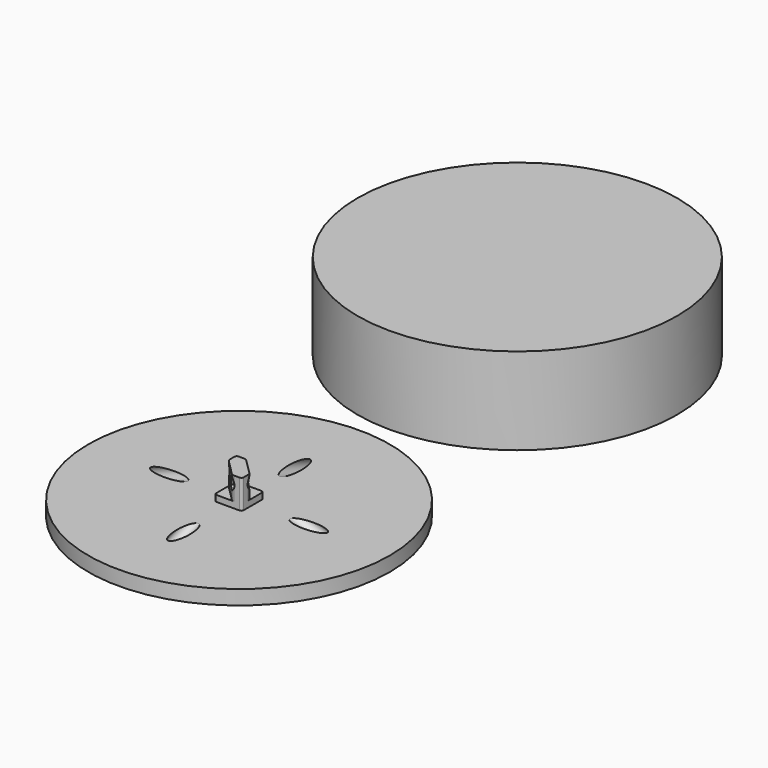
from build123d import *

# Parameters (mm, degrees)
F0_R              = 16.51
F1_DEPTH          = 1.5875
F2_W              = 3
F2_H              = 3
F3_DEPTH          = 3.175
F9_DEPTH          = 2.5
F10_R             = 17.5006
F11_DEPTH         = 9.525
F16_R             = 0.7
F17_DEPTH         = 1.27
F17_COPIES2_COUNT = 2
F18_DEPTH         = 25.4
F18_COPIES_COUNT  = 4
F19_R             = 0.254
F20_R             = 0.508


# Not quite as in the source:
# - a length typed as a fraction of an inch, garbled in the dataset ("3 / 203.2 mm" for 3/8 in), is restored
# - a pattern or mirror of a feature is missing from the dataset's text; its kind, count and spacing are read off the source's solid


with BuildPart() as f1:
    # F0 (on Top) → F1 (new body)
    with BuildSketch(Plane.XY):
        Circle(F0_R)
    extrude(amount=F1_DEPTH)

    # F2 (on face) → F3 (join)
    with BuildSketch(Plane.XY.offset(1.5875)):
        Rectangle(F2_W, F2_H)
    extrude(amount=F3_DEPTH)

    # F8 (on face) → F9 (cut)
    with BuildSketch(Plane.XY.offset(4.7625)):
        Polygon((-0.4393398282, 1.5), (1.5, -0.4393398282), (1.5, 1.5), align=None)
        Polygon((-1.5, -1.5), (0.4393398282, -1.5), (-1.5, 0.4393398282), align=None)
    extrude(amount=-F9_DEPTH, mode=Mode.SUBTRACT)


with BuildPart() as f11:
    # F10 (on Top) → F11 (new body)
    with BuildSketch(Plane.XY):
        with Locations((0, 38.1)):
            Circle(F10_R)
    extrude(amount=F11_DEPTH)

    # F12: cut F1
    add(f1.part, mode=Mode.SUBTRACT)


with BuildPart() as f1_1:
    add(f1.part)

    # F16 (on offset) → F17 (cut)
    with BuildSketch(Plane(origin=(0, -0.7814718533, -0.2844324935), x_dir=(-1, 0, 0), z_dir=(0, 0.9396926208, 0.3420201433))):
        with Locations((0, 4.102201201)):
            Circle(F16_R)
    f17 = extrude(amount=F17_DEPTH, mode=Mode.SUBTRACT)

    # F17_copies: F17 across plane
    add(f17.mirror(Plane(origin=(0, 0, 0), x_dir=(0.7071067812, 0.7071067812, 0), z_dir=(-0.7071067812, 0.7071067812, 0))), mode=Mode.SUBTRACT)

    # F17_copies1: F17 across plane
    add(f17.mirror(Plane(origin=(0, 0, 0), x_dir=(0.7071067812, -0.7071067812, 0), z_dir=(0.7071067812, 0.7071067812, 0))), mode=Mode.SUBTRACT)

    # F17_copies2: F17 ×2 about axis
    f17_copies2_axis = Axis((0, 0, 0), (0, 0, 1))
    for i in range(1, F17_COPIES2_COUNT):
        add(f17.rotate(f17_copies2_axis, i * 360 / F17_COPIES2_COUNT), mode=Mode.SUBTRACT)

    # F16 (on offset) → F18 (cut)
    with BuildSketch(Plane(origin=(0, -0.7814718533, -0.2844324935), x_dir=(-1, 0, 0), z_dir=(0, 0.9396926208, 0.3420201433))):
        with Locations((0, 4.102201201)):
            Circle(F16_R)
    f18 = extrude(amount=-F18_DEPTH, mode=Mode.SUBTRACT)

    # F18_copies: F18 ×4 about axis
    f18_copies_axis = Axis((0, 0, 0), (0, 0, 1))
    for i in range(1, F18_COPIES_COUNT):
        add(f18.rotate(f18_copies_axis, i * 360 / F18_COPIES_COUNT), mode=Mode.SUBTRACT)

    # F19
    f19_edges = [f1_1.edges().sort_by_distance(p)[0] for p in [
        (1.5, -1.5, 3.175),
        (-1.5, 1.5, 3.175),
        (1.5, 1.5, 1.925),
        (-1.5, -1.5, 1.925),
    ]]
    fillet(f19_edges, radius=F19_R)

    # F20
    f20_edges = [f1_1.edges().sort_by_distance(p)[0] for p in [
        (1.5, -0.43934, 2.751041),
        (1.5, -0.43934, 4.580975),
        (-0.43934, 1.5, 4.580975),
        (-0.43934, 1.5, 2.751041),
        (-1.5, 0.43934, 2.751041),
        (-1.5, 0.43934, 4.580975),
        (0.43934, -1.5, 2.751041),
        (0.43934, -1.5, 4.580975),
    ]]
    fillet(f20_edges, radius=F20_R)


solid = Compound([f11.part, f1_1.part])
